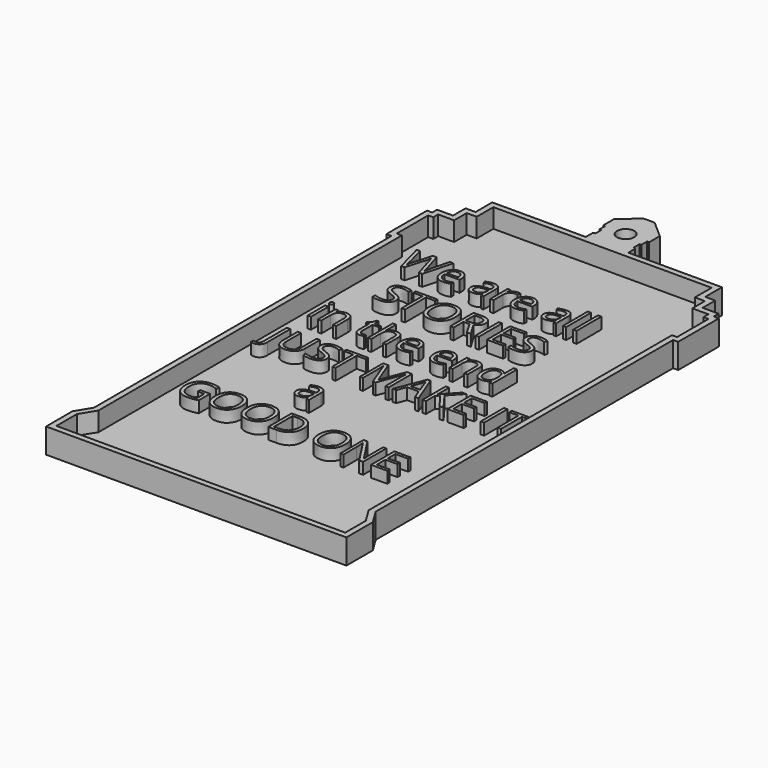
from build123d import *

# Parameters (mm, degrees)
F1_DEPTH     = 5
F2_T         = 1.5
F3_TEXT_SIZE = 10.6552692394
F4_DEPTH     = 3
F6_DEPTH     = 5
F8_D         = 4.5


# Not quite as in the source:
# - Text() gives the source's letters only with a copy of the font that has no kerning and outlines rounded to 1/6400 em; it was checked with that copy


with BuildPart() as f1:
    # F0 (on Top) → F1 (new body)
    with BuildSketch(Plane.XY):
        Polygon((0.8973410586, 73.7785175443), (0, 73.7785175443), (-0.8973410586, 73.7785175443), (-4.4930293225, 70.6085041165), (-4.4930293225, 69.2975744605), (-3.9780219086, 69.2975744605), (-3.9780219086, 67.4622729421), (-3.5004694946, 67.4622729421), (-3.5004694946, 63.4733140469), (-3.708244767, 63.1362199783), (-4.0640677325, 62.8927573562), (-4.0640677325, 60.0461736321), (-28.5353232175, 60.0461736321), (-28.5353232175, 54.5964986086), (-31.1457253993, 54.5964986086), (-31.1457253993, 50.4831373692), (-35.322368145, 50.4831373692), (-35.322368145, 48.885256052), (-36.6512984037, 48.885256052), (-36.6512984037, 38.6018566787), (-35.322368145, 38.6018566787), (-35.322368145, -60.5516731739), (-37.7688109875, -64.5384639502), (-37.7688109875, -71.2464079261), (0, -71.2464079261), (37.7688109875, -71.2464079261), (37.7688109875, -64.5384639502), (35.322368145, -60.5516731739), (35.322368145, 38.6018566787), (36.6512984037, 38.6018566787), (36.6512984037, 48.885256052), (35.322368145, 48.885256052), (35.322368145, 50.4831373692), (31.1457253993, 50.4831373692), (31.1457253993, 54.5964986086), (28.5353232175, 54.5964986086), (28.5353232175, 60.0461736321), (4.0640677325, 60.0461736321), (4.0640677325, 62.8927573562), (3.708244767, 63.1362199783), (3.5004694946, 63.4733140469), (3.5004694946, 67.4622729421), (3.9780219086, 67.4622729421), (3.9780219086, 69.2975744605), (4.4930293225, 69.2975744605), (4.4930293225, 70.6085041165), align=None)
    extrude(amount=F1_DEPTH)

    # F2
    f2_openings = [f1.faces().sort_by_distance(p)[0] for p in [
        (0, -5.683959, 5),
    ]]
    offset(amount=F2_T, openings=f2_openings, kind=Kind.INTERSECTION)

    # F3 (on face) → F4 (join)
    with BuildSketch(Plane.XY):
        with Locations((-31.5245579712, 30.9300628264)):
            Text('We are all', F3_TEXT_SIZE, font='Open Sans', text_align=(TextAlign.LEFT, TextAlign.BOTTOM))
        with Locations((-25.9871477384, 16.4388966608)):
            Text('STORIES', F3_TEXT_SIZE, font='Open Sans', text_align=(TextAlign.LEFT, TextAlign.BOTTOM))
        with Locations((-31.5245579712, 1.9477304953)):
            Text('in the end', F3_TEXT_SIZE, font='Open Sans', text_align=(TextAlign.LEFT, TextAlign.BOTTOM))
        with Locations((-31.5245579712, -12.5434356703)):
            Text('JUST MAKE IT', F3_TEXT_SIZE, font='Open Sans', text_align=(TextAlign.LEFT, TextAlign.BOTTOM))
        with Locations((-12.1436221563, -27.0346018358)):
            Text('a', F3_TEXT_SIZE, font='Open Sans', text_align=(TextAlign.LEFT, TextAlign.BOTTOM))
        with Locations((-31.5245579712, -41.5257680013)):
            Text('GOOD ONE', F3_TEXT_SIZE, font='Open Sans', text_align=(TextAlign.LEFT, TextAlign.BOTTOM))
    extrude(amount=F4_DEPTH)

    # F5 (on face) → F6 (join)
    with BuildSketch(Plane.XY):
        Polygon((0.8973410586, 73.7785175443), (0, 73.7785175443), (-0.8973410586, 73.7785175443), (-4.4930293225, 70.6085041165), (-4.4930293225, 69.2975744605), (-3.9780219086, 69.2975744605), (-3.9780219086, 67.4622729421), (-3.5004694946, 67.4622729421), (-3.5004694946, 63.4733140469), (-3.708244767, 63.1362199783), (-4.0640677325, 62.8927573562), (-4.0640677325, 60.0461736321), (4.0640677325, 60.0461736321), (4.0640677325, 62.8927573562), (3.708244767, 63.1362199783), (3.5004694946, 63.4733140469), (3.5004694946, 67.4622729421), (3.9780219086, 67.4622729421), (3.9780219086, 69.2975744605), (4.4930293225, 69.2975744605), (4.4930293225, 70.6085041165), align=None)
    extrude(amount=F6_DEPTH)

    # F8 (through all)
    with Locations(Plane.XY.offset(5)):
        with Locations((0, 67.6145404577)):
            Hole(F8_D / 2)


solid = f1.part
